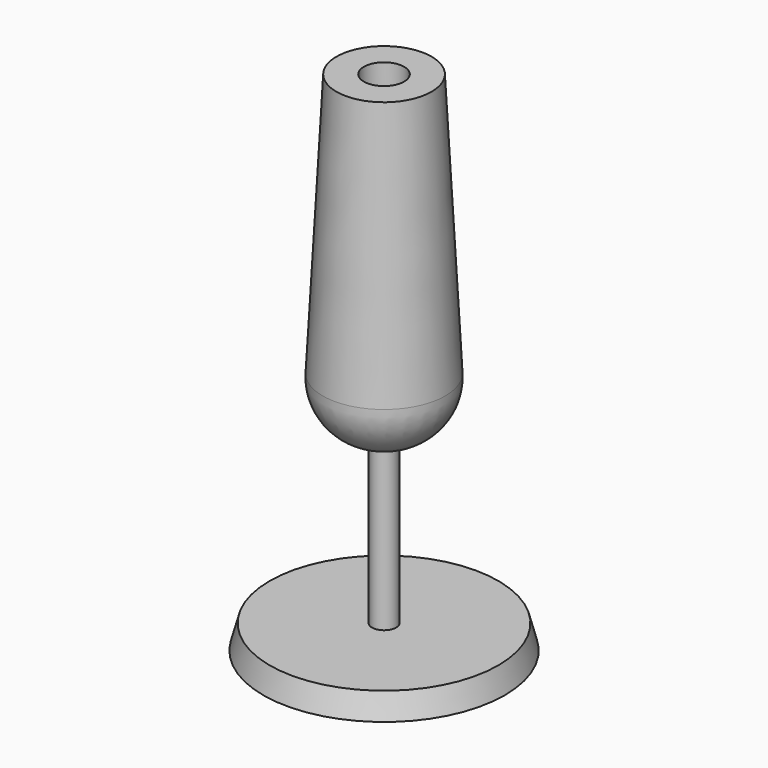
from build123d import *

# Parameters (mm, degrees)
F0_R     = 15
F1_DEPTH = 3
F1_TAPER = 15
F2_R     = 1.5
F3_DEPTH = 20
F4_R     = 8
F5_DEPTH = 40
F5_TAPER = 3
F6_R     = 2.5
F7_DEPTH = 5


# Not quite as in the source:
# - a fillet or chamfer that OpenCascade refuses, or shapes differently, is made with other operations: its cross-section is extruded or revolved along the edge and cut away or added


with BuildPart() as f1:
    # F0 (on Top) → F1 (new body)
    with BuildSketch(Plane.XY):
        Circle(F0_R)
    extrude(amount=F1_DEPTH, taper=F1_TAPER)

    # F2 (on face) → F3 (join)
    with BuildSketch(Plane.XY.offset(3)):
        Circle(F2_R)
    extrude(amount=F3_DEPTH)

    # F4 (on face) → F5 (join)
    with BuildSketch(Plane.XY.offset(23)):
        Circle(F4_R)
    extrude(amount=F5_DEPTH, taper=F5_TAPER)

    # F6 (on face) → F7 (cut)
    with BuildSketch(Plane.XY.offset(63)):
        Circle(F6_R)
    extrude(amount=-F7_DEPTH, mode=Mode.SUBTRACT)

    # F8: fillet of radius 7 on 1 edges, made by hand

    # F8_s1 → F8_t2 (revolve, cut)
    with BuildSketch(Plane.XZ):
        with BuildLine():
            ThreePointArc((1.5, 23), (5.9953541002, 25.4536811979), (7.6168139169, 30.3116260276))
            Line((7.6168139169, 30.3116260276), (8, 23))
            Line((8, 23), (1.5, 23))
        make_face()
    revolve(axis=Axis((0, 0, 23), (0, 0, -1)), mode=Mode.SUBTRACT)


solid = f1.part
